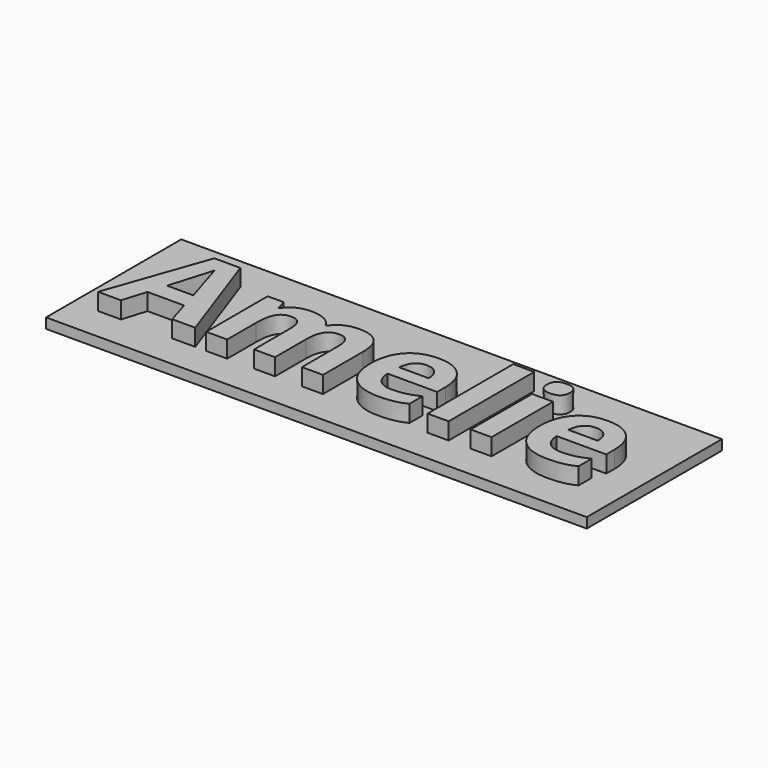
from build123d import *

# Parameters (mm, degrees)
F0_TEXT_SIZE = 41.6666666667
F1_DEPTH     = 8
F0_W         = 160
F0_H         = 50
F0_W_2       = 6.2044270833
F0_H_2       = 22.7473958333
F0_H_3       = 31.66015625
F2_DEPTH     = 3


# Not quite as in the source:
# - Text() gives the source's letters only with a copy of the font that has no kerning and outlines rounded to 1/6400 em; it was checked with that copy


with BuildPart() as f1:
    # F0 (on Top) → F1 (new body)
    with BuildSketch(Plane.XY):
        with Locations((-72.6171875, -15)):
            Text('Amelie', F0_TEXT_SIZE, font='Open Sans', font_style=FontStyle.BOLD, text_align=(TextAlign.LEFT, TextAlign.BOTTOM))
    extrude(amount=F1_DEPTH)


with BuildPart() as f2:
    # F0 (on Top) → F2 (new body)
    with BuildSketch(Plane.XY):
        Rectangle(F0_W, F0_H)
        Polygon((-43.8671875, -15), (-50.6640625, -15), (-52.8190104167, -7.9166666667), (-63.6653645833, -7.9166666667), (-65.8203125, -15), (-72.6171875, -15), (-62.1158854167, 14.8697916667), (-54.4075520833, 14.8697916667), align=None, mode=Mode.SUBTRACT)
        with BuildLine():
            Line((-20.2473958333, -3.5872395833), (-20.2473958333, -15))
            Line((-20.2473958333, -15), (-26.4518229167, -15))
            Line((-26.4518229167, -15), (-26.4518229167, -1.7122395833))
            add(Edge.make_bspline(
                [(-26.4518229167, -1.7122395833), (-26.4518229167, 0.7486979167), (-27.275390625, 1.9791666667)],
                knots=[0, 0, 0, 1, 1, 1], degree=2))
            add(Edge.make_bspline(
                [(-27.275390625, 1.9791666667), (-28.0989583333, 3.2096354167), (-29.8697916667, 3.2096354167)],
                knots=[0, 0, 0, 1, 1, 1], degree=2))
            add(Edge.make_bspline(
                [(-29.8697916667, 3.2096354167), (-32.2526041667, 3.2096354167), (-33.330078125, 1.4583333333)],
                knots=[0, 0, 0, 1, 1, 1], degree=2))
            add(Edge.make_bspline(
                [(-33.330078125, 1.4583333333), (-34.4075520833, -0.29296875), (-34.4075520833, -4.296875)],
                knots=[0, 0, 0, 1, 1, 1], degree=2))
            Line((-34.4075520833, -4.296875), (-34.4075520833, -15))
            Line((-34.4075520833, -15), (-40.6119791667, -15))
            Line((-40.6119791667, -15), (-40.6119791667, 7.7473958333))
            Line((-40.6119791667, 7.7473958333), (-35.8723958333, 7.7473958333))
            Line((-35.8723958333, 7.7473958333), (-35.0390625, 4.8372395833))
            Line((-35.0390625, 4.8372395833), (-34.6940104167, 4.8372395833))
            add(Edge.make_bspline(
                [(-34.6940104167, 4.8372395833), (-33.7760416667, 6.40625), (-32.0475260417, 7.2884114583)],
                knots=[0, 0, 0, 1, 1, 1], degree=2))
            add(Edge.make_bspline(
                [(-32.0475260417, 7.2884114583), (-30.3190104167, 8.1705729167), (-28.0794270833, 8.1705729167)],
                knots=[0, 0, 0, 1, 1, 1], degree=2))
            add(Edge.make_bspline(
                [(-28.0794270833, 8.1705729167), (-22.9752604167, 8.1705729167), (-21.1588541667, 4.8372395833)],
                knots=[0, 0, 0, 1, 1, 1], degree=2))
            Line((-21.1588541667, 4.8372395833), (-20.6119791667, 4.8372395833))
            add(Edge.make_bspline(
                [(-20.6119791667, 4.8372395833), (-19.6940104167, 6.42578125), (-17.9166666667, 7.2981770833)],
                knots=[0, 0, 0, 1, 1, 1], degree=2))
            add(Edge.make_bspline(
                [(-17.9166666667, 7.2981770833), (-16.1393229167, 8.1705729167), (-13.8997395833, 8.1705729167)],
                knots=[0, 0, 0, 1, 1, 1], degree=2))
            add(Edge.make_bspline(
                [(-13.8997395833, 8.1705729167), (-10.0325520833, 8.1705729167), (-8.0501302083, 6.1881510417)],
                knots=[0, 0, 0, 1, 1, 1], degree=2))
            add(Edge.make_bspline(
                [(-8.0501302083, 6.1881510417), (-6.0677083333, 4.2057291667), (-6.0677083333, -0.1692708333)],
                knots=[0, 0, 0, 1, 1, 1], degree=2))
            Line((-6.0677083333, -0.1692708333), (-6.0677083333, -15))
            Line((-6.0677083333, -15), (-12.2916666667, -15))
            Line((-12.2916666667, -15), (-12.2916666667, -1.7122395833))
            add(Edge.make_bspline(
                [(-12.2916666667, -1.7122395833), (-12.2916666667, 0.7486979167), (-13.115234375, 1.9791666667)],
                knots=[0, 0, 0, 1, 1, 1], degree=2))
            add(Edge.make_bspline(
                [(-13.115234375, 1.9791666667), (-13.9388020833, 3.2096354167), (-15.7096354167, 3.2096354167)],
                knots=[0, 0, 0, 1, 1, 1], degree=2))
            add(Edge.make_bspline(
                [(-15.7096354167, 3.2096354167), (-17.98828125, 3.2096354167), (-19.1178385417, 1.58203125)],
                knots=[0, 0, 0, 1, 1, 1], degree=2))
            add(Edge.make_bspline(
                [(-19.1178385417, 1.58203125), (-20.2473958333, -0.0455729167), (-20.2473958333, -3.5872395833)],
                knots=[0, 0, 0, 1, 1, 1], degree=2))
        make_face(mode=Mode.SUBTRACT)
        with BuildLine():
            add(Edge.make_bspline(
                [(15.1106770833, -15.0130208333), (13.26171875, -15.41015625), (10.5924479167, -15.41015625)],
                knots=[0, 0, 0, 1, 1, 1], degree=2))
            add(Edge.make_bspline(
                [(10.5924479167, -15.41015625), (5.1041666667, -15.41015625), (2.01171875, -12.3763020833)],
                knots=[0, 0, 0, 1, 1, 1], degree=2))
            add(Edge.make_bspline(
                [(2.01171875, -12.3763020833), (-1.0807291667, -9.3424479167), (-1.0807291667, -3.7890625)],
                knots=[0, 0, 0, 1, 1, 1], degree=2))
            add(Edge.make_bspline(
                [(-1.0807291667, -3.7890625), (-1.0807291667, 1.9270833333), (1.77734375, 5.048828125)],
                knots=[0, 0, 0, 1, 1, 1], degree=2))
            add(Edge.make_bspline(
                [(1.77734375, 5.048828125), (4.6354166667, 8.1705729167), (9.6809895833, 8.1705729167)],
                knots=[0, 0, 0, 1, 1, 1], degree=2))
            add(Edge.make_bspline(
                [(9.6809895833, 8.1705729167), (14.4986979167, 8.1705729167), (17.1842447917, 5.4264322917)],
                knots=[0, 0, 0, 1, 1, 1], degree=2))
            add(Edge.make_bspline(
                [(17.1842447917, 5.4264322917), (19.8697916667, 2.6822916667), (19.8697916667, -2.1614583333)],
                knots=[0, 0, 0, 1, 1, 1], degree=2))
            Line((19.8697916667, -2.1614583333), (19.8697916667, -5.17578125))
            Line((19.8697916667, -5.17578125), (5.2018229167, -5.17578125))
            add(Edge.make_bspline(
                [(5.2018229167, -5.17578125), (5.3059895833, -7.8190104167), (6.7708333333, -9.3033854167)],
                knots=[0, 0, 0, 1, 1, 1], degree=2))
            add(Edge.make_bspline(
                [(6.7708333333, -9.3033854167), (8.2356770833, -10.7877604167), (10.87890625, -10.7877604167)],
                knots=[0, 0, 0, 1, 1, 1], degree=2))
            add(Edge.make_bspline(
                [(10.87890625, -10.7877604167), (12.9361979167, -10.7877604167), (14.765625, -10.361328125)],
                knots=[0, 0, 0, 1, 1, 1], degree=2))
            add(Edge.make_bspline(
                [(14.765625, -10.361328125), (16.5950520833, -9.9348958333), (18.5872395833, -8.9973958333)],
                knots=[0, 0, 0, 1, 1, 1], degree=2))
            Line((18.5872395833, -8.9973958333), (18.5872395833, -13.8020833333))
            add(Edge.make_bspline(
                [(18.5872395833, -13.8020833333), (16.9596354167, -14.6158854167), (15.1106770833, -15.0130208333)],
                knots=[0, 0, 0, 1, 1, 1], degree=2))
        make_face(mode=Mode.SUBTRACT)
        with Locations((40.732421875, -3.6263020833)):
            Rectangle(F0_W_2, F0_H_2, mode=Mode.SUBTRACT)
        with BuildLine():
            add(Edge.make_bspline(
                [(65.15625, -15.0130208333), (63.3072916667, -15.41015625), (60.6380208333, -15.41015625)],
                knots=[0, 0, 0, 1, 1, 1], degree=2))
            add(Edge.make_bspline(
                [(60.6380208333, -15.41015625), (55.1497395833, -15.41015625), (52.0572916667, -12.3763020833)],
                knots=[0, 0, 0, 1, 1, 1], degree=2))
            add(Edge.make_bspline(
                [(52.0572916667, -12.3763020833), (48.96484375, -9.3424479167), (48.96484375, -3.7890625)],
                knots=[0, 0, 0, 1, 1, 1], degree=2))
            add(Edge.make_bspline(
                [(48.96484375, -3.7890625), (48.96484375, 1.9270833333), (51.8229166667, 5.048828125)],
                knots=[0, 0, 0, 1, 1, 1], degree=2))
            add(Edge.make_bspline(
                [(51.8229166667, 5.048828125), (54.6809895833, 8.1705729167), (59.7265625, 8.1705729167)],
                knots=[0, 0, 0, 1, 1, 1], degree=2))
            add(Edge.make_bspline(
                [(59.7265625, 8.1705729167), (64.5442708333, 8.1705729167), (67.2298177083, 5.4264322917)],
                knots=[0, 0, 0, 1, 1, 1], degree=2))
            add(Edge.make_bspline(
                [(67.2298177083, 5.4264322917), (69.9153645833, 2.6822916667), (69.9153645833, -2.1614583333)],
                knots=[0, 0, 0, 1, 1, 1], degree=2))
            Line((69.9153645833, -2.1614583333), (69.9153645833, -5.17578125))
            Line((69.9153645833, -5.17578125), (55.2473958333, -5.17578125))
            add(Edge.make_bspline(
                [(55.2473958333, -5.17578125), (55.3515625, -7.8190104167), (56.81640625, -9.3033854167)],
                knots=[0, 0, 0, 1, 1, 1], degree=2))
            add(Edge.make_bspline(
                [(56.81640625, -9.3033854167), (58.28125, -10.7877604167), (60.9244791667, -10.7877604167)],
                knots=[0, 0, 0, 1, 1, 1], degree=2))
            add(Edge.make_bspline(
                [(60.9244791667, -10.7877604167), (62.9817708333, -10.7877604167), (64.8111979167, -10.361328125)],
                knots=[0, 0, 0, 1, 1, 1], degree=2))
            add(Edge.make_bspline(
                [(64.8111979167, -10.361328125), (66.640625, -9.9348958333), (68.6328125, -8.9973958333)],
                knots=[0, 0, 0, 1, 1, 1], degree=2))
            Line((68.6328125, -8.9973958333), (68.6328125, -13.8020833333))
            add(Edge.make_bspline(
                [(68.6328125, -13.8020833333), (67.0052083333, -14.6158854167), (65.15625, -15.0130208333)],
                knots=[0, 0, 0, 1, 1, 1], degree=2))
        make_face(mode=Mode.SUBTRACT)
        with Locations((28.017578125, 0.830078125)):
            Rectangle(F0_W_2, F0_H_3, mode=Mode.SUBTRACT)
        with BuildLine():
            add(Edge.make_bspline(
                [(40.7421875, 10.5729166667), (37.36328125, 10.5729166667), (37.36328125, 13.6263020833)],
                knots=[0, 0, 0, 1, 1, 1], degree=2))
            add(Edge.make_bspline(
                [(37.36328125, 13.6263020833), (37.36328125, 16.66015625), (40.7421875, 16.66015625)],
                knots=[0, 0, 0, 1, 1, 1], degree=2))
            add(Edge.make_bspline(
                [(40.7421875, 16.66015625), (44.12109375, 16.66015625), (44.12109375, 13.6263020833)],
                knots=[0, 0, 0, 1, 1, 1], degree=2))
            add(Edge.make_bspline(
                [(44.12109375, 13.6263020833), (44.12109375, 12.1809895833), (43.2779947917, 11.376953125)],
                knots=[0, 0, 0, 1, 1, 1], degree=2))
            add(Edge.make_bspline(
                [(43.2779947917, 11.376953125), (42.4348958333, 10.5729166667), (40.7421875, 10.5729166667)],
                knots=[0, 0, 0, 1, 1, 1], degree=2))
        make_face(mode=Mode.SUBTRACT)
    extrude(amount=F2_DEPTH)


with BuildPart() as f2b:
    # F0 (on Top) → F2, piece 2 (new body)
    with BuildSketch(Plane.XY):
        with BuildLine():
            Line((-62.0768229167, -2.6302083333), (-54.3294270833, -2.6302083333))
            add(Edge.make_bspline(
                [(-54.3294270833, -2.6302083333), (-57.3177083333, 6.9921875), (-57.6953125, 8.2552083333)],
                knots=[0, 0, 0, 1, 1, 1], degree=2))
            add(Edge.make_bspline(
                [(-57.6953125, 8.2552083333), (-58.0729166667, 9.5182291667), (-58.2356770833, 10.2473958333)],
                knots=[0, 0, 0, 1, 1, 1], degree=2))
            add(Edge.make_bspline(
                [(-58.2356770833, 10.2473958333), (-58.90625, 7.6432291667), (-62.0768229167, -2.6302083333)],
                knots=[0, 0, 0, 1, 1, 1], degree=2))
        make_face()
    extrude(amount=F2_DEPTH)


with BuildPart() as f2c:
    # F0 (on Top) → F2, piece 3 (new body)
    with BuildSketch(Plane.XY):
        with BuildLine():
            add(Edge.make_bspline(
                [(12.8515625, 2.5065104167), (11.6927083333, 3.7565104167), (9.7200520833, 3.7565104167)],
                knots=[0, 0, 0, 1, 1, 1], degree=2))
            add(Edge.make_bspline(
                [(9.7200520833, 3.7565104167), (7.7473958333, 3.7565104167), (6.6276041667, 2.5065104167)],
                knots=[0, 0, 0, 1, 1, 1], degree=2))
            add(Edge.make_bspline(
                [(6.6276041667, 2.5065104167), (5.5078125, 1.2565104167), (5.3450520833, -1.0416666667)],
                knots=[0, 0, 0, 1, 1, 1], degree=2))
            Line((5.3450520833, -1.0416666667), (14.0559895833, -1.0416666667))
            add(Edge.make_bspline(
                [(14.0559895833, -1.0416666667), (14.0104166667, 1.2565104167), (12.8515625, 2.5065104167)],
                knots=[0, 0, 0, 1, 1, 1], degree=2))
        make_face()
    extrude(amount=F2_DEPTH)


with BuildPart() as f2d:
    # F0 (on Top) → F2, piece 4 (new body)
    with BuildSketch(Plane.XY):
        with BuildLine():
            add(Edge.make_bspline(
                [(62.8971354167, 2.5065104167), (61.73828125, 3.7565104167), (59.765625, 3.7565104167)],
                knots=[0, 0, 0, 1, 1, 1], degree=2))
            add(Edge.make_bspline(
                [(59.765625, 3.7565104167), (57.79296875, 3.7565104167), (56.6731770833, 2.5065104167)],
                knots=[0, 0, 0, 1, 1, 1], degree=2))
            add(Edge.make_bspline(
                [(56.6731770833, 2.5065104167), (55.5533854167, 1.2565104167), (55.390625, -1.0416666667)],
                knots=[0, 0, 0, 1, 1, 1], degree=2))
            Line((55.390625, -1.0416666667), (64.1015625, -1.0416666667))
            add(Edge.make_bspline(
                [(64.1015625, -1.0416666667), (64.0559895833, 1.2565104167), (62.8971354167, 2.5065104167)],
                knots=[0, 0, 0, 1, 1, 1], degree=2))
        make_face()
    extrude(amount=F2_DEPTH)


solid = Compound([f1.part, f2.part, f2b.part, f2c.part, f2d.part])
